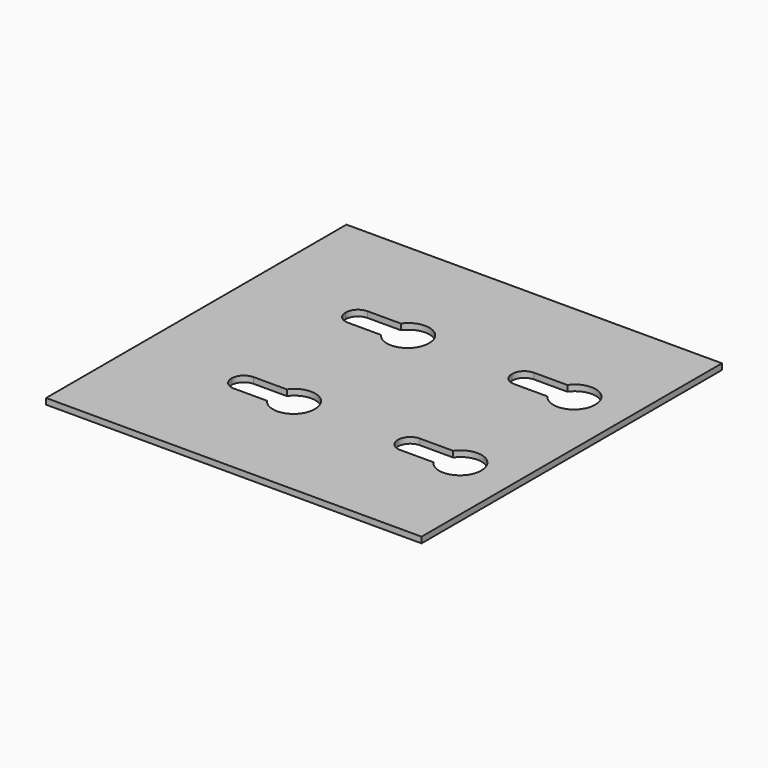
from build123d import *

# Parameters (mm, degrees)
F0_W     = 200.66
F0_H     = 200.66
F1_DEPTH = 3.175


# Not quite as in the source:
# - a length typed as a fraction of an inch, garbled in the dataset ("3 / 203.2 mm" for 3/8 in), is restored


with BuildPart() as f1:
    # F0 (on Top) → F1 (new body)
    with BuildSketch(Plane.XY):
        Rectangle(F0_W, F0_H)
        with BuildLine():
            Line((-6.4755703305, -37.973), (-6.4755703305, -38.227))
            ThreePointArc((-6.4755703305, -38.227), (-14.2002143688, -48.9498629888), (-26.715108043, -44.704))
            Line((-26.715108043, -44.704), (-30.0367761716, -44.704))
            Line((-30.0367761716, -44.704), (-44.4783061624, -44.704))
            ThreePointArc((-44.4783061624, -44.704), (-49.0582367841, -42.8069306217), (-50.9553061624, -38.227))
            Line((-50.9553061624, -38.227), (-50.9553061624, -37.973))
            ThreePointArc((-50.9553061624, -37.973), (-49.0582367841, -33.3930693783), (-44.4783061624, -31.496))
            Line((-44.4783061624, -31.496), (-30.0367761716, -31.496))
            Line((-30.0367761716, -31.496), (-26.715108043, -31.496))
            ThreePointArc((-26.715108043, -31.496), (-14.2002143688, -27.2501370112), (-6.4755703305, -37.973))
        make_face(mode=Mode.SUBTRACT)
        with BuildLine():
            Line((82.4244296695, -37.973), (82.4244296695, -38.227))
            ThreePointArc((82.4244296695, -38.227), (74.6997856312, -48.9498629888), (62.184891957, -44.704))
            Line((62.184891957, -44.704), (58.8632238284, -44.704))
            Line((58.8632238284, -44.704), (44.4216938376, -44.704))
            ThreePointArc((44.4216938376, -44.704), (39.8417632159, -42.8069306217), (37.9446938376, -38.227))
            Line((37.9446938376, -38.227), (37.9446938376, -37.973))
            ThreePointArc((37.9446938376, -37.973), (39.8417632159, -33.3930693783), (44.4216938376, -31.496))
            Line((44.4216938376, -31.496), (58.8632238284, -31.496))
            Line((58.8632238284, -31.496), (62.184891957, -31.496))
            ThreePointArc((62.184891957, -31.496), (74.6997856312, -27.2501370112), (82.4244296695, -37.973))
        make_face(mode=Mode.SUBTRACT)
        with BuildLine():
            ThreePointArc((-50.9553061624, 38.227), (-49.0582367841, 42.8069306217), (-44.4783061624, 44.704))
            Line((-44.4783061624, 44.704), (-30.0367761716, 44.704))
            Line((-30.0367761716, 44.704), (-26.715108043, 44.704))
            ThreePointArc((-26.715108043, 44.704), (-14.2002143688, 48.9498629888), (-6.4755703305, 38.227))
            Line((-6.4755703305, 38.227), (-6.4755703305, 37.973))
            ThreePointArc((-6.4755703305, 37.973), (-14.2002143688, 27.2501370112), (-26.715108043, 31.496))
            Line((-26.715108043, 31.496), (-30.0367761716, 31.496))
            Line((-30.0367761716, 31.496), (-44.4783061624, 31.496))
            ThreePointArc((-44.4783061624, 31.496), (-49.0582367841, 33.3930693783), (-50.9553061624, 37.973))
            Line((-50.9553061624, 37.973), (-50.9553061624, 38.227))
        make_face(mode=Mode.SUBTRACT)
        with BuildLine():
            Line((82.4244296695, 38.227), (82.4244296695, 37.973))
            ThreePointArc((82.4244296695, 37.973), (74.6997856312, 27.2501370112), (62.184891957, 31.496))
            Line((62.184891957, 31.496), (58.8632238284, 31.496))
            Line((58.8632238284, 31.496), (44.4216938376, 31.496))
            ThreePointArc((44.4216938376, 31.496), (39.8417632159, 33.3930693783), (37.9446938376, 37.973))
            Line((37.9446938376, 37.973), (37.9446938376, 38.227))
            ThreePointArc((37.9446938376, 38.227), (39.8417632159, 42.8069306217), (44.4216938376, 44.704))
            Line((44.4216938376, 44.704), (58.8632238284, 44.704))
            Line((58.8632238284, 44.704), (62.184891957, 44.704))
            ThreePointArc((62.184891957, 44.704), (74.6997856312, 48.9498629888), (82.4244296695, 38.227))
        make_face(mode=Mode.SUBTRACT)
    extrude(amount=F1_DEPTH)


solid = f1.part
